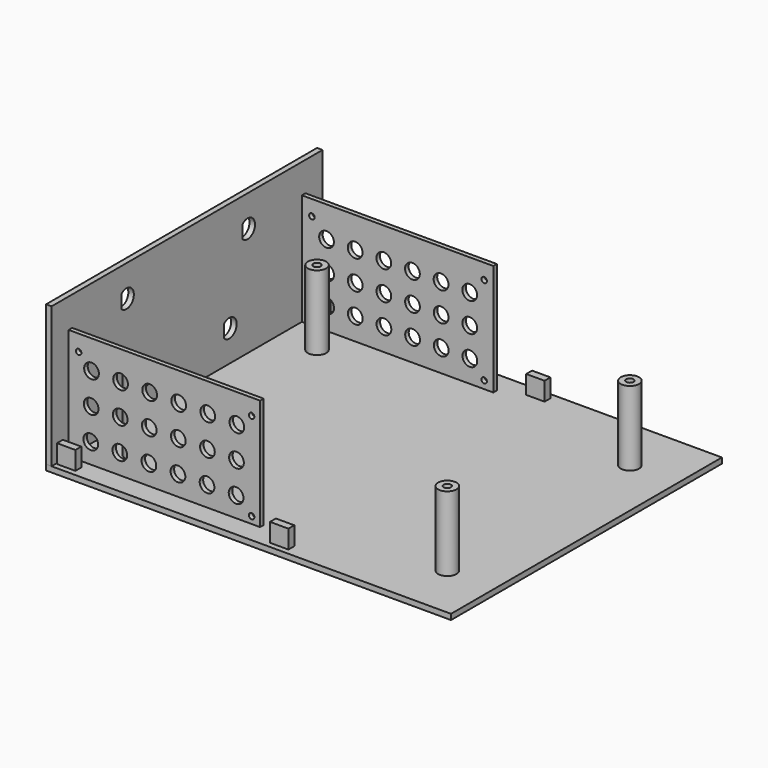
from build123d import *

# Parameters (mm, degrees)
F0_R      = 2.5
F0_R_2    = 1
F1_DEPTH  = 21
F2_DEPTH  = 39
F0_W      = 52
F0_H      = 1.2
F3_DEPTH  = 31
F4_R      = 0.75
F4_R_2    = 2.0049588284
F5_DEPTH  = 25
F6_R      = 0.75
F6_R_2    = 2
F7_DEPTH  = 25
F8_DEPTH  = 0.75
F10_DEPTH = 25
F11_W     = 5
F11_H     = 2
F12_DEPTH = 5


# Not quite as in the source:
# - a feature names something its author has since deleted; it is built from what else it names


with BuildPart() as f1:
    # F0 (on Top) → F1 (new body)
    with BuildSketch(Plane.XY):
        with Locations((-43, 31)):
            Circle(F0_R)
        with Locations((-43, 31)):
            Circle(F0_R_2, mode=Mode.SUBTRACT)
    extrude(amount=F1_DEPTH)


with BuildPart() as f1b:
    # F0 (on Top) → F1, piece 2 (new body)
    with BuildSketch(Plane.XY):
        with Locations((-43, -31)):
            Circle(F0_R)
        with Locations((-43, -31)):
            Circle(F0_R_2, mode=Mode.SUBTRACT)
    extrude(amount=F1_DEPTH)


with BuildPart() as f1c:
    # F0 (on Top) → F1, piece 3 (new body)
    with BuildSketch(Plane.XY):
        with Locations((42, -31)):
            Circle(F0_R)
        with Locations((42, -31)):
            Circle(F0_R_2, mode=Mode.SUBTRACT)
    extrude(amount=F1_DEPTH)


with BuildPart() as f1d:
    # F0 (on Top) → F1, piece 4 (new body)
    with BuildSketch(Plane.XY):
        with Locations((42, 31)):
            Circle(F0_R)
        with Locations((42, 31)):
            Circle(F0_R_2, mode=Mode.SUBTRACT)
    extrude(amount=F1_DEPTH)


with BuildPart() as f2:
    # F0 (on Top) → F2 (new body)
    with BuildSketch(Plane.XY):
        Polygon((-53.5, 46), (-55, 46), (-55, -46), (-53.5, -46), (-53.5, -40.2), (-53.5, -39), (-53.5, 39), (-53.5, 40.2), align=None)
    extrude(amount=F2_DEPTH)

    # F0 (on Top) → F3 (join)
    with BuildSketch(Plane.XY):
        with Locations((-27.5, 39.6)):
            Rectangle(F0_W, F0_H)
        with Locations((-27.5, -39.6)):
            Rectangle(F0_W, F0_H)
    extrude(amount=F3_DEPTH)

    # F4 (on face) → F5 (cut)
    with BuildSketch(Plane(origin=(0, 40.2, 0), x_dir=(-1, 0, 0), z_dir=(0, 1, 0))):
        with Locations((4, 26.8378742281)):
            Circle(F4_R)
        with Locations((50.8, 26.8378742281)):
            Circle(F4_R)
        with Locations((50.8, 2.8378742281)):
            Circle(F4_R)
        with Locations((4, 2.8378742281)):
            Circle(F4_R)
        with Locations((7.9205203801, 22.5936546922)):
            Circle(F4_R_2)
        with Locations((7.9, 14.7)):
            Circle(F4_R_2)
        with Locations((7.8794796199, 6.8063453078)):
            Circle(F4_R_2)
        with Locations((15.7, 22.6)):
            Circle(F4_R_2)
        with Locations((15.6794796199, 14.7063453078)):
            Circle(F4_R_2)
        with Locations((15.6589592397, 6.8126906157)):
            Circle(F4_R_2)
        with Locations((23.4794796199, 22.6063453078)):
            Circle(F4_R_2)
        with Locations((23.4589592397, 14.7126906157)):
            Circle(F4_R_2)
        with Locations((23.4384388596, 6.8190359235)):
            Circle(F4_R_2)
        with Locations((31.2589592397, 22.6126906157)):
            Circle(F4_R_2)
        with Locations((31.2384388596, 14.7190359235)):
            Circle(F4_R_2)
        with Locations((31.2179184794, 6.8253812313)):
            Circle(F4_R_2)
        with Locations((39.0384388596, 22.6190359235)):
            Circle(F4_R_2)
        with Locations((39.0179184794, 14.7253812313)):
            Circle(F4_R_2)
        with Locations((38.9973980993, 6.8317265391)):
            Circle(F4_R_2)
        with Locations((46.8179184794, 22.6253812313)):
            Circle(F4_R_2)
        with Locations((46.7973980993, 14.7317265391)):
            Circle(F4_R_2)
        with Locations((46.7768777192, 6.838071847)):
            Circle(F4_R_2)
    extrude(amount=-F5_DEPTH, mode=Mode.SUBTRACT)

    # F6 (on face) → F7 (cut)
    with BuildSketch(Plane.XZ.offset(40.2)):
        with Locations((-50.799280405, 26.6274153497)):
            Circle(F6_R)
        with Locations((-3.799280405, 26.6274153497)):
            Circle(F6_R)
        with Locations((-3.799280405, 2.6274153497)):
            Circle(F6_R)
        with Locations((-50.799280405, 2.6274153497)):
            Circle(F6_R)
        with Locations((-47.2966842353, 23.1979489326)):
            Circle(F6_R_2)
        with Locations((-47.4, 14.7)):
            Circle(F6_R_2)
        with Locations((-47.5033157647, 6.2020510674)):
            Circle(F6_R_2)
        with Locations((-39.4, 23.2)):
            Circle(F6_R_2)
        with Locations((-39.5033157647, 14.7020510674)):
            Circle(F6_R_2)
        with Locations((-39.6066315293, 6.2041021347)):
            Circle(F6_R_2)
        with Locations((-31.5033157647, 23.2020510674)):
            Circle(F6_R_2)
        with Locations((-31.6066315293, 14.7041021347)):
            Circle(F6_R_2)
        with Locations((-31.709947294, 6.2061532021)):
            Circle(F6_R_2)
        with Locations((-23.6066315293, 23.2041021347)):
            Circle(F6_R_2)
        with Locations((-23.709947294, 14.7061532021)):
            Circle(F6_R_2)
        with Locations((-23.8132630587, 6.2082042694)):
            Circle(F6_R_2)
        with Locations((-15.709947294, 23.2061532021)):
            Circle(F6_R_2)
        with Locations((-15.8132630587, 14.7082042694)):
            Circle(F6_R_2)
        with Locations((-15.9165788233, 6.2102553368)):
            Circle(F6_R_2)
        with Locations((-7.8132630587, 23.2082042694)):
            Circle(F6_R_2)
        with Locations((-7.9165788233, 14.7102553368)):
            Circle(F6_R_2)
        with Locations((-8.019894588, 6.2123064041)):
            Circle(F6_R_2)
    extrude(amount=-F7_DEPTH, mode=Mode.SUBTRACT)

    # F9 (on face) → F10 (cut)
    with BuildSketch(Plane(origin=(-55, 0, 0), x_dir=(0, -1, 0), z_dir=(-1, 0, 0))):
        with BuildLine():
            Line((-18.8740566373, 28.6679799402), (-18.8740566373, 32.3320200598))
            ThreePointArc((-18.8740566373, 32.3320200598), (-23.0751452595, 30.5), (-18.8740566373, 28.6679799402))
        make_face()
        with BuildLine():
            Line((22.2670137882, 28.6594617957), (22.2670137882, 32.3405382043))
            ThreePointArc((22.2670137882, 32.3405382043), (18.0751452595, 30.5), (22.2670137882, 28.6594617957))
        make_face()
        with BuildLine():
            Line((-12.5011904165, 7.5581133879), (-12.5011904165, 10.9418866121))
            ThreePointArc((-12.5011904165, 10.9418866121), (-16.841711998, 9.25), (-12.5011904165, 7.5581133879))
        make_face()
        with BuildLine():
            Line((16.1892920732, 7.5658242771), (16.1892920732, 10.9341757229))
            ThreePointArc((16.1892920732, 10.9341757229), (11.841711998, 9.25), (16.1892920732, 7.5658242771))
        make_face()
    extrude(amount=-F10_DEPTH, mode=Mode.SUBTRACT)


with BuildPart() as f8:
    # F0 (on Top) → F8 (new body, symmetric)
    with BuildSketch(Plane.XY):
        Polygon((-53.5, 46), (-55, 46), (-55, -46), (-53.5, -46), (-53.5, -40.2), (-53.5, -39), (-53.5, 39), (-53.5, 40.2), align=None)
        Polygon((55, 46), (-53.5, 46), (-53.5, 40.2), (-1.5, 40.2), (-1.5, 39), (-53.5, 39), (-53.5, -39), (-1.5, -39), (-1.5, -40.2), (-53.5, -40.2), (-53.5, -46), (55, -46), align=None)
        with Locations((-43, -31)):
            Circle(F0_R, mode=Mode.SUBTRACT)
        with Locations((42, -31)):
            Circle(F0_R, mode=Mode.SUBTRACT)
        with Locations((-43, 31)):
            Circle(F0_R, mode=Mode.SUBTRACT)
        with Locations((42, 31)):
            Circle(F0_R, mode=Mode.SUBTRACT)
    extrude(amount=F8_DEPTH, both=True)


with BuildPart() as f12:
    # F11 (on face) → F12 (new body)
    with BuildSketch(Plane.XY.offset(0.75)):
        with Locations((7.1263094991, -43.5)):
            Rectangle(F11_W, F11_H)
    extrude(amount=F12_DEPTH)


with BuildPart() as f12b:
    # F11 (on face) → F12, piece 2 (new body)
    with BuildSketch(Plane.XY.offset(0.75)):
        with Locations((7.1263094991, 43.5)):
            Rectangle(F11_W, F11_H)
    extrude(amount=F12_DEPTH)


with BuildPart() as f12c:
    # F11 (on face) → F12, piece 3 (new body)
    with BuildSketch(Plane.XY.offset(0.75)):
        with Locations((-51, 43.5)):
            Rectangle(F11_W, F11_H)
    extrude(amount=F12_DEPTH)


with BuildPart() as f12d:
    # F11 (on face) → F12, piece 4 (new body)
    with BuildSketch(Plane.XY.offset(0.75)):
        with Locations((-50.7398670912, -43.5)):
            Rectangle(F11_W, F11_H)
    extrude(amount=F12_DEPTH)


solid = Compound([f1.part, f1b.part, f1c.part, f1d.part, f2.part, f8.part, f12.part, f12b.part, f12c.part, f12d.part])
